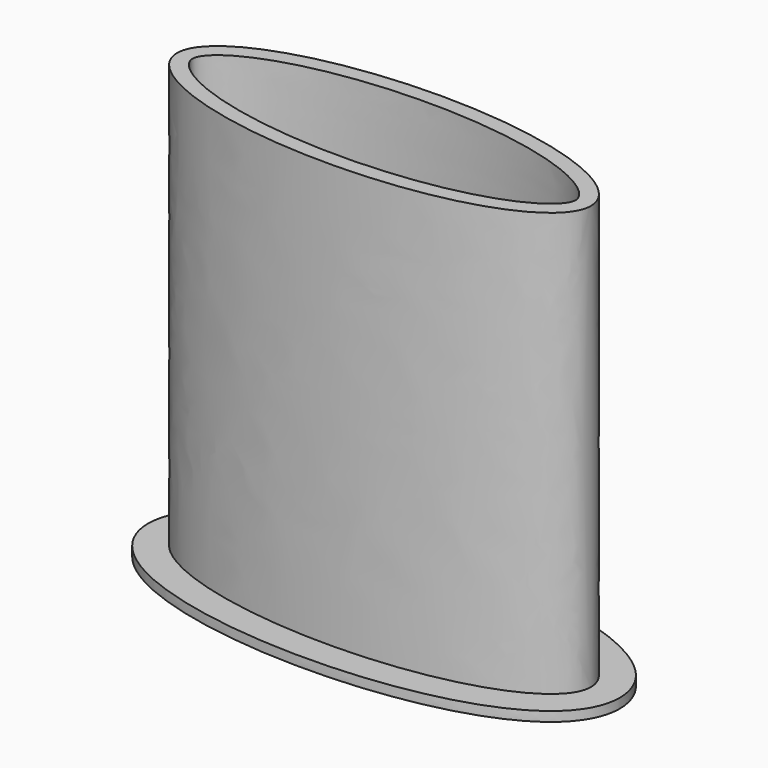
from build123d import *

# Parameters (mm, degrees)
F1_DEPTH = 1
F2_DEPTH = 45


# Not quite as in the source:
# - the dataset's text gives a spline's control points without its knots; the knots are read off the source's solid


with BuildPart() as f1:
    # F0 (on Top) → F1 (new body)
    with BuildSketch(Plane.XY):
        with BuildLine():
            add(Edge.make_bspline(
                [(24.5, 0), (24.5, 0.2646472108), (24.4622521814, 0.7939416324), (24.2433856506, 1.8179546827), (23.733966274, 2.9877638714), (22.8686760106, 4.1741116895), (21.8245873438, 5.1838507173), (20.6274468303, 6.063126892), (18.8347151616, 7.1024910688), (16.2729130204, 8.1817657734), (13.3010271943, 9.0316907534), (10.694938898, 9.57643936), (7.9840165454, 10.0229369254), (5.1427729266, 10.3229002696), (2.2219201086, 10.4744575494), (0, 10.5127712253), (-2.2219201086, 10.4744575494), (-5.1427729266, 10.3229002696), (-7.9840165454, 10.0229369254), (-10.694938898, 9.57643936), (-13.3010271943, 9.0316907534), (-16.2729130204, 8.1817657734), (-18.8347151616, 7.1024910688), (-20.6274468303, 6.063126892), (-21.8245873438, 5.1838507173), (-22.8686760106, 4.1741116895), (-23.733966274, 2.9877638714), (-24.2433856506, 1.8179546827), (-24.4622521814, 0.7939416324), (-24.5188739093, 0), (-24.4622521814, -0.7939416324), (-24.2433856506, -1.8179546827), (-23.733966274, -2.9877638714), (-22.8686760106, -4.1741116895), (-21.8245873438, -5.1838507173), (-20.6274468303, -6.063126892), (-18.8347151616, -7.1024910688), (-16.2729130204, -8.1817657734), (-13.3010271943, -9.0316907534), (-10.694938898, -9.57643936), (-7.9840165454, -10.0229369254), (-5.1427729266, -10.3229002696), (-2.2219201086, -10.4744575494), (0, -10.5127712253), (2.2219201086, -10.4744575494), (5.1427729266, -10.3229002696), (7.9840165454, -10.0229369254), (10.694938898, -9.57643936), (13.3010271943, -9.0316907534), (16.2729130204, -8.1817657734), (18.8347151616, -7.1024910688), (20.6274468303, -6.063126892), (21.8245873438, -5.1838507173), (22.8686760106, -4.1741116895), (23.733966274, -2.9877638714), (24.2433856506, -1.8179546827), (24.4622521814, -0.7939416324), (24.5, -0.2646472108), (24.5, 0)],
                knots=[0, 0, 0, 0, 0.0078125, 0.015625, 0.03125, 0.046875, 0.0625, 0.078125, 0.09375, 0.125, 0.15625, 0.171875, 0.1875, 0.21875, 0.234375, 0.25, 0.265625, 0.28125, 0.3125, 0.328125, 0.34375, 0.375, 0.40625, 0.421875, 0.4375, 0.453125, 0.46875, 0.484375, 0.4921875, 0.5, 0.5078125, 0.515625, 0.53125, 0.546875, 0.5625, 0.578125, 0.59375, 0.625, 0.65625, 0.671875, 0.6875, 0.71875, 0.734375, 0.75, 0.765625, 0.78125, 0.8125, 0.828125, 0.84375, 0.875, 0.90625, 0.921875, 0.9375, 0.953125, 0.96875, 0.984375, 0.9921875, 1, 1, 1, 1], degree=3))
        make_face()
        with BuildLine():
            add(Edge.make_bspline(
                [(21.5, 0), (21.5, 12.9903810568), (-10.75, 6.4951905284), (-43, 0), (-10.75, -6.4951905284), (21.5, -12.9903810568), (21.5, 0)],
                knots=[0, 0, 0, 2.0943951024, 2.0943951024, 4.1887902048, 4.1887902048, 6.2831853072, 6.2831853072, 6.2831853072], degree=2, weights=[1, 0.5, 1, 0.5, 1, 0.5, 1]))
        make_face(mode=Mode.SUBTRACT)
    extrude(amount=F1_DEPTH)

    # F0 (on Top) → F2 (join)
    with BuildSketch(Plane.XY):
        with BuildLine():
            add(Edge.make_bspline(
                [(21.5, 0), (21.5, 12.9903810568), (-10.75, 6.4951905284), (-43, 0), (-10.75, -6.4951905284), (21.5, -12.9903810568), (21.5, 0)],
                knots=[0, 0, 0, 2.0943951024, 2.0943951024, 4.1887902048, 4.1887902048, 6.2831853072, 6.2831853072, 6.2831853072], degree=2, weights=[1, 0.5, 1, 0.5, 1, 0.5, 1]))
        make_face()
        with BuildLine():
            add(Edge.make_bspline(
                [(19.8999997228, 0), (19.8999997228, 0.0959871973), (19.8751027733, 0.2879615919), (19.7255909098, 0.655936407), (19.4018331813, 1.1162725747), (18.8704647794, 1.6396704204), (18.1234990745, 2.1938313377), (16.8449758406, 2.9397570408), (14.7805298062, 3.8199106698), (12.1923561061, 4.5633846105), (9.8548405952, 5.0523819706), (7.3902672306, 5.4586337415), (4.7715889929, 5.7357218815), (2.063779282, 5.8762585586), (0, 5.911870305), (-2.063779282, 5.8762585586), (-4.7715889929, 5.7357218815), (-7.3902672306, 5.4586337415), (-9.8548405952, 5.0523819706), (-12.1923561061, 4.5633846105), (-14.7805298062, 3.8199106698), (-16.8449758406, 2.9397570408), (-18.1234990745, 2.1938313377), (-18.8704647794, 1.6396704204), (-19.4018331813, 1.1162725747), (-19.7255909098, 0.655936407), (-19.8751027733, 0.2879615919), (-19.9124481976, 0), (-19.8751027733, -0.2879615919), (-19.7255909098, -0.655936407), (-19.4018331813, -1.1162725747), (-18.8704647794, -1.6396704204), (-18.1234990745, -2.1938313377), (-16.8449758406, -2.9397570408), (-14.7805298062, -3.8199106698), (-12.1923561061, -4.5633846105), (-9.8548405952, -5.0523819706), (-7.3902672306, -5.4586337415), (-4.7715889929, -5.7357218815), (-2.063779282, -5.8762585586), (0, -5.911870305), (2.063779282, -5.8762585586), (4.7715889929, -5.7357218815), (7.3902672306, -5.4586337415), (9.8548405952, -5.0523819706), (12.1923561061, -4.5633846105), (14.7805298062, -3.8199106698), (16.8449758406, -2.9397570408), (18.1234990745, -2.1938313377), (18.8704647794, -1.6396704204), (19.4018331813, -1.1162725747), (19.7255909098, -0.655936407), (19.8751027733, -0.2879615919), (19.8999997228, -0.0959871973), (19.8999997228, 0)],
                knots=[0, 0, 0, 0, 0.015625, 0.03125, 0.046875, 0.0625, 0.078125, 0.09375, 0.125, 0.15625, 0.171875, 0.1875, 0.21875, 0.234375, 0.25, 0.265625, 0.28125, 0.3125, 0.328125, 0.34375, 0.375, 0.40625, 0.421875, 0.4375, 0.453125, 0.46875, 0.484375, 0.5, 0.515625, 0.53125, 0.546875, 0.5625, 0.578125, 0.59375, 0.625, 0.65625, 0.671875, 0.6875, 0.71875, 0.734375, 0.75, 0.765625, 0.78125, 0.8125, 0.828125, 0.84375, 0.875, 0.90625, 0.921875, 0.9375, 0.953125, 0.96875, 0.984375, 1, 1, 1, 1], degree=3))
        make_face(mode=Mode.SUBTRACT)
    extrude(amount=F2_DEPTH)


solid = f1.part
